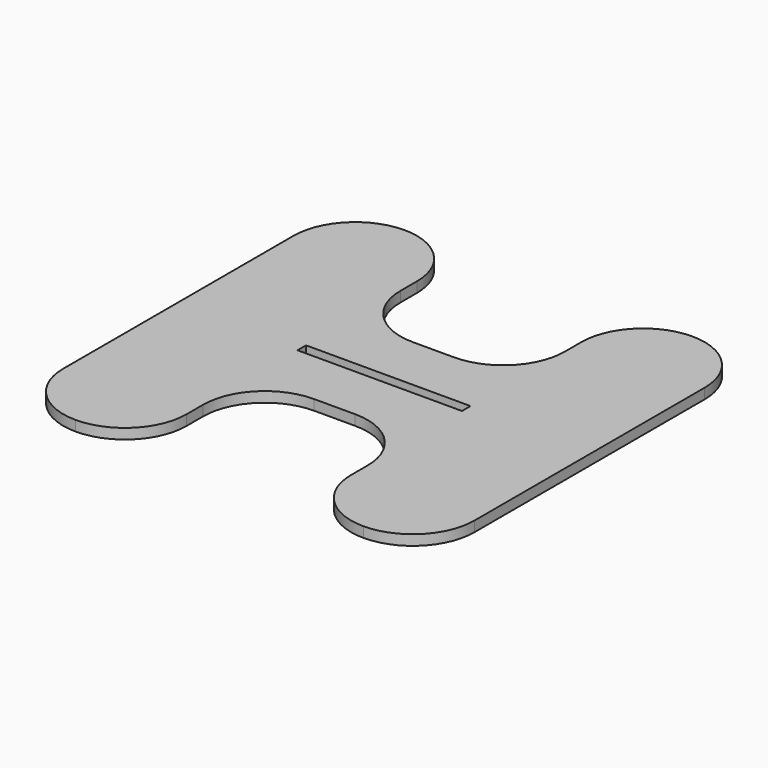
from build123d import *

# Parameters (mm, degrees)
F0_W     = 50.8
F0_H     = 3.302
F1_DEPTH = 3.175
F2_R     = 19.04999


# Not quite as in the source:
# - a fillet or chamfer is up to 0.001 mm smaller than in the source, because OpenCascade refuses the exact size


with BuildPart() as f1:
    # F0 (on Top) → F1 (new body)
    with BuildSketch(Plane.XY):
        Polygon((18.769003178, 68.6352171788), (-19.330996822, 68.6352171788), (-19.330996822, -58.3647828212), (18.769003178, -58.3647828212), (18.769003178, -13.9147828212), (69.569003178, -13.9147828212), (69.569003178, -58.3647828212), (107.669003178, -58.3647828212), (107.669003178, 68.6352171788), (69.569003178, 68.6352171788), (69.569003178, 24.1852171788), (18.769003178, 24.1852171788), align=None)
        with Locations((44.169003178, 5.1352171788)):
            Rectangle(F0_W, F0_H, mode=Mode.SUBTRACT)
    extrude(amount=F1_DEPTH)

    # F2 (radius 19.05 in the source; OpenCascade refuses exactly that, so slightly less here)
    f2_edges = [f1.edges().sort_by_distance(p)[0] for p in [
        (18.769003, -58.364783, 1.5875),
        (-19.330997, -58.364783, 1.5875),
        (69.569003, -58.364783, 1.5875),
        (107.669003, -58.364783, 1.5875),
        (18.769003, -13.914783, 1.5875),
        (69.569003, -13.914783, 1.5875),
        (-19.330997, 68.635217, 1.5875),
        (18.769003, 68.635217, 1.5875),
        (69.569003, 24.185217, 1.5875),
        (69.569003, 68.635217, 1.5875),
        (107.669003, 68.635217, 1.5875),
        (18.769003, 24.185217, 1.5875),
    ]]
    fillet(f2_edges, radius=F2_R)


solid = f1.part
